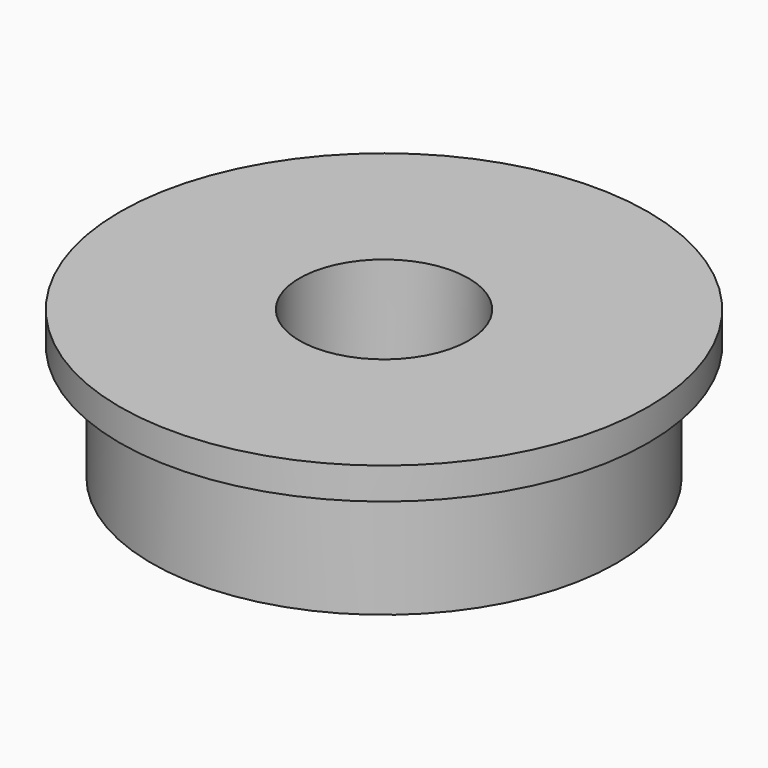
from build123d import *


with BuildPart() as f1:
    # F0 (on Front) → F1 (revolve)
    with BuildSketch(Plane.XZ):
        Polygon((4, 7), (4, 0), (11, 0), (11, 5.5), (12.5, 5.5), (12.5, 7), align=None)
    revolve(axis=Axis((0, 0, 3.7551978178), (0, 0, 1)))


solid = f1.part
